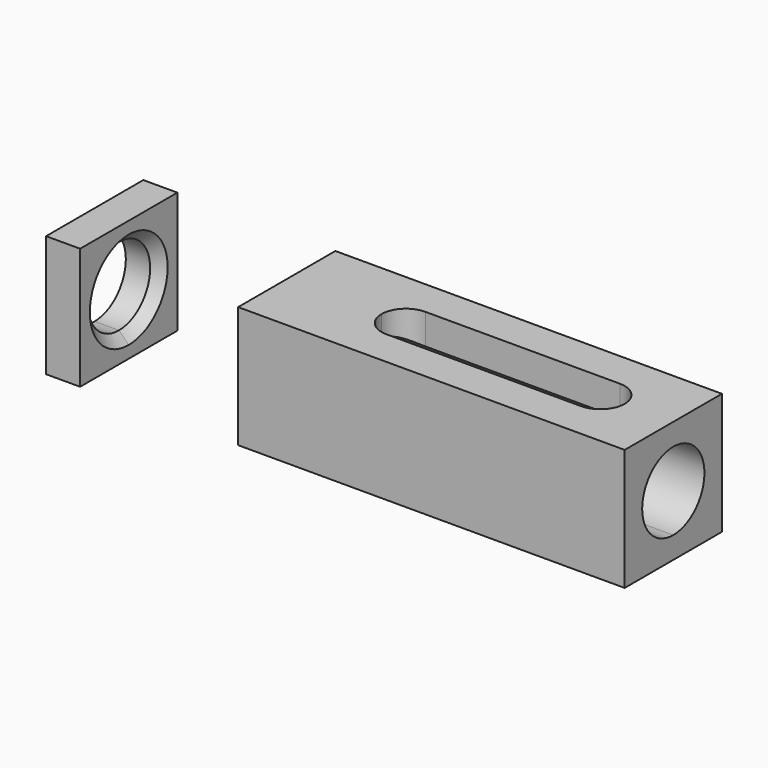
from build123d import *

# Parameters (mm, degrees)
F0_W     = 119
F0_H     = 25
F1_DEPTH = 25
F3_DEPTH = 119.001
F4_W     = 32.5
F4_H     = 25
F5_DEPTH = 25.001
F6_SIZE  = 2
F7_W     = 50
F7_H     = 5
F8_DEPTH = 10
F9_R     = 4.9999
F10_R    = 4.9999


# Not quite as in the source:
# - a fillet or chamfer is up to 0.001 mm smaller than in the source, because OpenCascade refuses the exact size


with BuildPart() as f1:
    # F0 (on Top) → F1 (new body)
    with BuildSketch(Plane.XY):
        Rectangle(F0_W, F0_H)
    extrude(amount=F1_DEPTH)

    # F2 (on face) → F3 (cut, through all)
    with BuildSketch(Plane(origin=(-59.5, 0, 0), x_dir=(0, -1, 0), z_dir=(-1, 0, 0))):
        with BuildLine():
            ThreePointArc((8, 12.5), (5.6568542495, 18.1568542495), (0, 20.5))
            Line((0, 20.5), (0, 4.5))
            ThreePointArc((0, 4.5), (5.6568542495, 6.8431457505), (8, 12.5))
        make_face()
        with BuildLine():
            Line((0, 4.5), (0, 20.5))
            ThreePointArc((0, 20.5), (-8, 12.5), (0, 4.5))
        make_face()
    extrude(amount=-F3_DEPTH, mode=Mode.SUBTRACT)

    # F4 (on face) → F5 (cut, through all)
    with BuildSketch(Plane.XY.offset(25)):
        with Locations((-36.25, 0)):
            Rectangle(F4_W, F4_H)
    extrude(amount=-F5_DEPTH, mode=Mode.SUBTRACT)

    # F6
    f6_edges = [f1.edges().sort_by_distance(p)[0] for p in [
        (-52.5, 8, 12.5),
    ]]
    chamfer(f6_edges, length=F6_SIZE)

    # F7 (on face) → F8 (cut)
    with BuildSketch(Plane.XY.offset(25)):
        with Locations((24.5, 2.5)):
            Rectangle(F7_W, F7_H)
        with Locations((24.5, -2.5)):
            Rectangle(F7_W, F7_H)
    extrude(amount=-F8_DEPTH, mode=Mode.SUBTRACT)

    # F9 (radius 5 in the source; OpenCascade refuses exactly that, so slightly less here)
    f9_edges = [f1.edges().sort_by_distance(p)[0] for p in [
        (-0.5, 5, 21.872499),
        (-0.5, -5, 21.872499),
    ]]
    fillet(f9_edges, radius=F9_R)

    # F10 (radius 5 in the source; OpenCascade refuses exactly that, so slightly less here)
    f10_edges = [f1.edges().sort_by_distance(p)[0] for p in [
        (49.5, 5, 21.872499),
        (49.5, -5, 21.872499),
    ]]
    fillet(f10_edges, radius=F10_R)


solid = f1.part
